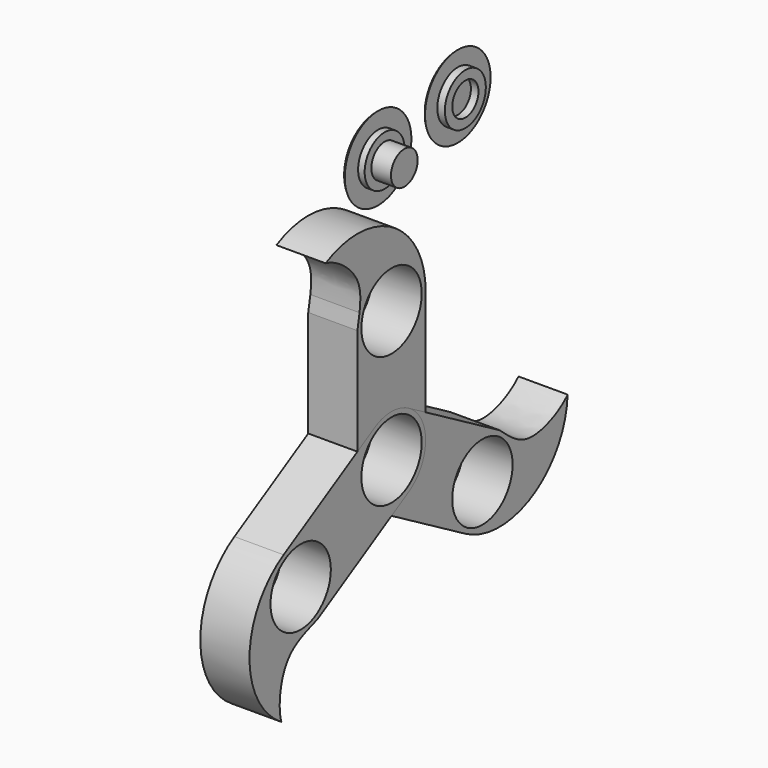
from build123d import *

# Parameters (mm, degrees)
F1_DEPTH  = 15
F2_COUNT  = 3
F3_R      = 12.7
F3_R_2    = 7.62
F4_DEPTH  = 2
F3_R_3    = 5.08
F5_DEPTH  = 4
F6_DEPTH  = 10
F8_R      = 12.5
F8_R_2    = 7.8074571386
F9_DEPTH  = 1.7
F8_R_3    = 5
F10_DEPTH = 4
F11_DEPTH = 1.7


# Not quite as in the source:
# - a fillet or chamfer that OpenCascade refuses, or shapes differently, is made with other operations: its cross-section is extruded or revolved along the edge and cut away or added


with BuildPart() as f1:
    # F0 (on Right) → F1 (new body)
    with BuildSketch(Plane.YZ):
        with BuildLine():
            ThreePointArc((-25.2000448819, 22.8609375315), (-10.7197131173, 31.1695194223), (0, 18.3710706205))
            ThreePointArc((0, 18.3710706205), (-12.5693121356, 40.6335193512), (-38.124355653, 41.3710706205))
            add(Edge.make_bspline(
                [(-38.124355653, 41.3710706205), (-33.870069896, 40.4348456264), (-24.5113742969, 33.6690367859), (-24.7364824739, 25.9636118629), (-25.2000448819, 22.8609375315)],
                knots=[0, 0, 0, 0, 0.5176076193, 0.8448578002, 0.8448578002, 0.8448578002, 0.8448578002], degree=3))
        make_face()
        with BuildLine():
            ThreePointArc((-24.5, 18.3710706205), (-13, 29.8710706205), (-1.5, 18.3710706205))
            Line((-1.5, 18.3710706205), (0, 18.3710706205))
            ThreePointArc((0, 18.3710706205), (-10.7197131173, 31.1695194223), (-25.2000448819, 22.8609375315))
            add(Edge.make_bspline(
                [(-25.2000448819, 22.8609375315), (-25.4198097466, 21.3900270506), (-25.7241634459, 19.8925897433), (-26, 18.3710706205)],
                knots=[0.8448578002, 0.8448578002, 0.8448578002, 0.8448578002, 1, 1, 1, 1], degree=3))
            Line((-26, 18.3710706205), (-24.5, 18.3710706205))
        make_face()
        with BuildLine():
            Line((0, 18.3710706205), (-1.5, 18.3710706205))
            ThreePointArc((-1.5, 18.3710706205), (-13, 6.8710706205), (-24.5, 18.3710706205))
            Line((-24.5, 18.3710706205), (-26, 18.3710706205))
            ThreePointArc((-26, 18.3710706205), (-13, 5.3710706205), (0, 18.3710706205))
        make_face()
        with BuildLine():
            ThreePointArc((-26, -7.6289293795), (-7.6152236891, -0.0137056904), (0, 18.3710706205))
            ThreePointArc((0, 18.3710706205), (-13, 5.3710706205), (-26, 18.3710706205))
            Line((-26, 18.3710706205), (-26, -7.6289293795))
        make_face()
        with BuildLine():
            Line((0, -21.6289293795), (0, 18.3710706205))
            ThreePointArc((0, 18.3710706205), (-7.6152236891, -0.0137056904), (-26, -7.6289293795))
            Line((-26, -7.6289293795), (-26, -21.6289293795))
            ThreePointArc((-26, -21.6289293795), (-13, -8.6289293795), (0, -21.6289293795))
        make_face()
        with BuildLine():
            ThreePointArc((-26, -21.6289293795), (-13, -34.6289293795), (0, -21.6289293795))
            Line((0, -21.6289293795), (-1.5, -21.6289293795))
            ThreePointArc((-1.5, -21.6289293795), (-13, -33.1289293795), (-24.5, -21.6289293795))
            Line((-24.5, -21.6289293795), (-26, -21.6289293795))
        make_face()
        with BuildLine():
            Line((-1.5, -21.6289293795), (0, -21.6289293795))
            ThreePointArc((0, -21.6289293795), (-13, -8.6289293795), (-26, -21.6289293795))
            Line((-26, -21.6289293795), (-24.5, -21.6289293795))
            ThreePointArc((-24.5, -21.6289293795), (-13, -10.1289293795), (-1.5, -21.6289293795))
        make_face()
    extrude(amount=F1_DEPTH)


with BuildPart() as f2_1:
    # F2: instance of F1
    add(f1.part.rotate(Axis((0, -13, -21.6289293795), (-1, 0, 0)), 1 * 360 / F2_COUNT))


with BuildPart() as f2_2:
    # F2: instance of F1
    add(f1.part.rotate(Axis((0, -13, -21.6289293795), (-1, 0, 0)), 2 * 360 / F2_COUNT))


with BuildPart() as f4:
    # F3 (on Right) → F4 (new body)
    with BuildSketch(Plane.YZ):
        with Locations((-1.8790969625, 50.6367385387)):
            Circle(F3_R)
        with Locations((-1.8790969625, 50.6367385387)):
            Circle(F3_R_2, mode=Mode.SUBTRACT)
    extrude(amount=F4_DEPTH)

    # F3 (on Right) → F5 (join)
    with BuildSketch(Plane.YZ):
        with Locations((-1.8790969625, 50.6367385387)):
            Circle(F3_R_2)
        with Locations((-1.8790969625, 50.6367385387)):
            Circle(F3_R_3, mode=Mode.SUBTRACT)
    extrude(amount=F5_DEPTH)

    # F3 (on Right) → F6 (join)
    with BuildSketch(Plane.YZ):
        with Locations((-1.8790969625, 50.6367385387)):
            Circle(F3_R_3)
    extrude(amount=F6_DEPTH)

    # F7: fillet of radius 5.08 on 1 edges, made by hand

    # F7_s1 → F7_t2 (revolve, cut)
    with BuildSketch(Plane.XY.offset(50.6367385387)):
        with BuildLine():
            ThreePointArc((2, 10.8209030375), (0.5273743839, 9.0349865961), (0, 6.7811010621))
            Line((0, 6.7811010621), (0, 10.8209030375))
            Line((0, 10.8209030375), (2, 10.8209030375))
        make_face()
    revolve(axis=Axis((0, -1.8790969625, 50.6367385387), (1, 0, 0)), mode=Mode.SUBTRACT)


with BuildPart() as f9:
    # F8 (on Right) → F9 (new body)
    with BuildSketch(Plane.YZ):
        with Locations((28.8851223886, 54.6414889395)):
            Circle(F8_R)
        with Locations((28.8851223886, 54.6414889395)):
            Circle(F8_R_2, mode=Mode.SUBTRACT)
    extrude(amount=F9_DEPTH)

    # F8 (on Right) → F10 (join)
    with BuildSketch(Plane.YZ):
        with Locations((28.8851223886, 54.6414889395)):
            Circle(F8_R_2)
        with Locations((28.8851223886, 54.6414889395)):
            Circle(F8_R_3, mode=Mode.SUBTRACT)
    extrude(amount=F10_DEPTH)

    # F8 (on Right) → F11 (join)
    with BuildSketch(Plane.YZ):
        with Locations((28.8851223886, 54.6414889395)):
            Circle(F8_R_3)
    extrude(amount=F11_DEPTH)

    # F12: fillet of radius 5 on 1 edges, made by hand

    # F12_s1 → F12_t2 (revolve, cut)
    with BuildSketch(Plane.XY.offset(54.6414889395)):
        with BuildLine():
            ThreePointArc((1.7, 41.3851223886), (0.4447832104, 39.6903472072), (0, 37.6287943944))
            Line((0, 37.6287943944), (0, 41.3851223886))
            Line((0, 41.3851223886), (1.7, 41.3851223886))
        make_face()
    revolve(axis=Axis((0, 28.8851223886, 54.6414889395), (1, 0, 0)), mode=Mode.SUBTRACT)


solid = Compound([f1.part, f2_1.part, f2_2.part, f4.part, f9.part])
